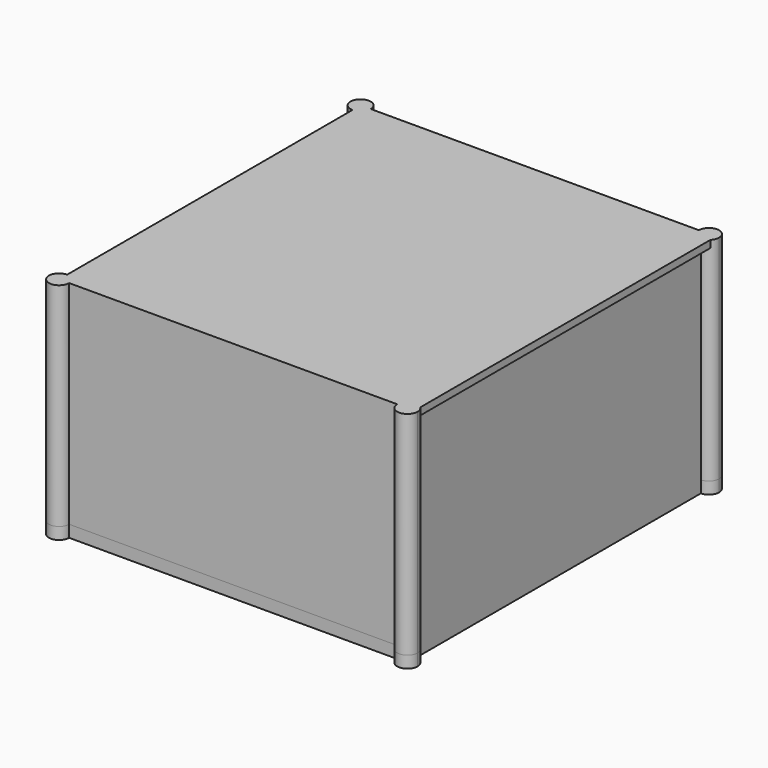
from build123d import *

# Parameters (mm, degrees)
F0_W          = 5
F0_H          = 26
F1_DEPTH      = 5
F2_DEPTH      = 86
F3_DEPTH      = 3
F4_DEPTH      = 89
F5_START      = 86
F5_DEPTH      = 3
F6_R          = 1.925
F7_DEPTH      = 20
F7_DEPTH_BACK = 5
F8_DEPTH      = 3
F9_DEPTH      = 1.2426406871
F10_DEPTH     = 1.2426406871


# Not quite as in the source:
# - a feature names something its author has since deleted; it is built from what else it names


with BuildPart() as f1:
    # F0 (on Top) → F1 (new body)
    with BuildSketch(Plane.XY):
        with BuildLine():
            ThreePointArc((73, 74.7573593129), (71.3764116996, 75.0803111054), (70, 76))
            Line((70, 76), (70, -76))
            ThreePointArc((70, -76), (71.3764116996, -75.0803111054), (73, -74.7573593129))
            Line((73, -74.7573593129), (73, 74.7573593129))
        make_face()
        Polygon((70, -76), (70, 76), (-30, 76), (-30, 50), (-30, -50), (-30, -76), align=None)
        Polygon((-35, 50), (-35, 76), (-70, 76), (-70, -76), (-35, -76), (-35, -50), (-30, -50), (-30, 50), align=None)
        with Locations((-32.5, -63)):
            Rectangle(F0_W, F0_H)
        with Locations((-32.5, 63)):
            Rectangle(F0_W, F0_H)
        with BuildLine():
            Line((-70, -76), (-70, 76))
            ThreePointArc((-70, 76), (-71.3764116996, 75.0803111054), (-73, 74.7573593129))
            Line((-73, 74.7573593129), (-73, -74.7573593129))
            ThreePointArc((-73, -74.7573593129), (-71.3764116996, -75.0803111054), (-70, -76))
        make_face()
        with BuildLine():
            ThreePointArc((73, -74.7573593129), (71.3764116996, -75.0803111054), (70, -76))
            Line((70, -76), (73, -76))
            Line((73, -76), (73, -74.7573593129))
        make_face()
        with BuildLine():
            Line((73, -76), (70, -76))
            ThreePointArc((70, -76), (69.0803111054, -77.3764116996), (68.7573593129, -79))
            Line((68.7573593129, -79), (73, -79))
            Line((73, -79), (73, -76))
        make_face()
        with BuildLine():
            Line((73, -74.7573593129), (73, -76))
            Line((73, -76), (73, -79))
            Line((73, -79), (68.7573593129, -79))
            ThreePointArc((68.7573593129, -79), (73, -83.2426406871), (77.2426406871, -79))
            ThreePointArc((77.2426406871, -79), (76, -76), (73, -74.7573593129))
        make_face()
        with BuildLine():
            Line((73, 76), (70, 76))
            ThreePointArc((70, 76), (71.3764116996, 75.0803111054), (73, 74.7573593129))
            Line((73, 74.7573593129), (73, 76))
        make_face()
        with BuildLine():
            ThreePointArc((68.7573593129, 79), (69.0803111054, 77.3764116996), (70, 76))
            Line((70, 76), (73, 76))
            Line((73, 76), (73, 79))
            Line((73, 79), (68.7573593129, 79))
        make_face()
        with BuildLine():
            Line((73, 79), (73, 76))
            Line((73, 76), (73, 74.7573593129))
            ThreePointArc((73, 74.7573593129), (76, 76), (77.2426406871, 79))
            ThreePointArc((77.2426406871, 79), (73, 83.2426406871), (68.7573593129, 79))
            Line((68.7573593129, 79), (73, 79))
        make_face()
        with BuildLine():
            Line((-30, 76), (70, 76))
            ThreePointArc((70, 76), (69.0803111054, 77.3764116996), (68.7573593129, 79))
            Line((68.7573593129, 79), (-68.7573593129, 79))
            ThreePointArc((-68.7573593129, 79), (-69.0803111054, 77.3764116996), (-70, 76))
            Line((-70, 76), (-35, 76))
            Line((-35, 76), (-30, 76))
        make_face()
        with BuildLine():
            ThreePointArc((-70, 76), (-69.0803111054, 77.3764116996), (-68.7573593129, 79))
            Line((-68.7573593129, 79), (-73, 79))
            Line((-73, 79), (-73, 74.7573593129))
            ThreePointArc((-73, 74.7573593129), (-71.3764116996, 75.0803111054), (-70, 76))
        make_face()
        with BuildLine():
            Line((-73, 79), (-68.7573593129, 79))
            ThreePointArc((-68.7573593129, 79), (-76, 82), (-73, 74.7573593129))
            Line((-73, 74.7573593129), (-73, 79))
        make_face()
        with BuildLine():
            Line((-73, -79), (-68.7573593129, -79))
            ThreePointArc((-68.7573593129, -79), (-69.0803111054, -77.3764116996), (-70, -76))
            ThreePointArc((-70, -76), (-71.3764116996, -75.0803111054), (-73, -74.7573593129))
            Line((-73, -74.7573593129), (-73, -79))
        make_face()
        with BuildLine():
            ThreePointArc((-73, -74.7573593129), (-76, -82), (-68.7573593129, -79))
            Line((-68.7573593129, -79), (-73, -79))
            Line((-73, -79), (-73, -74.7573593129))
        make_face()
        with BuildLine():
            ThreePointArc((68.7573593129, -79), (69.0803111054, -77.3764116996), (70, -76))
            Line((70, -76), (-30, -76))
            Line((-30, -76), (-35, -76))
            Line((-35, -76), (-70, -76))
            ThreePointArc((-70, -76), (-69.0803111054, -77.3764116996), (-68.7573593129, -79))
            Line((-68.7573593129, -79), (68.7573593129, -79))
        make_face()
    extrude(amount=-F1_DEPTH)

    # F0 (on Top) → F2 (join)
    with BuildSketch(Plane.XY):
        with BuildLine():
            ThreePointArc((73, 74.7573593129), (71.3764116996, 75.0803111054), (70, 76))
            Line((70, 76), (70, -76))
            ThreePointArc((70, -76), (71.3764116996, -75.0803111054), (73, -74.7573593129))
            Line((73, -74.7573593129), (73, 74.7573593129))
        make_face()
    extrude(amount=F2_DEPTH)

    # F0 (on Top) → F3 (join)
    with BuildSketch(Plane.XY):
        with Locations((-32.5, 63)):
            Rectangle(F0_W, F0_H)
        with Locations((-32.5, -63)):
            Rectangle(F0_W, F0_H)
    extrude(amount=F3_DEPTH)


with BuildPart() as f4:
    # F0 (on Top) → F4 (new body)
    with BuildSketch(Plane.XY):
        with BuildLine():
            Line((-70, -76), (-70, 76))
            ThreePointArc((-70, 76), (-71.3764116996, 75.0803111054), (-73, 74.7573593129))
            Line((-73, 74.7573593129), (-73, -74.7573593129))
            ThreePointArc((-73, -74.7573593129), (-71.3764116996, -75.0803111054), (-70, -76))
        make_face()
        with BuildLine():
            Line((73, -76), (70, -76))
            ThreePointArc((70, -76), (69.0803111054, -77.3764116996), (68.7573593129, -79))
            Line((68.7573593129, -79), (73, -79))
            Line((73, -79), (73, -76))
        make_face()
        with BuildLine():
            ThreePointArc((68.7573593129, 79), (69.0803111054, 77.3764116996), (70, 76))
            Line((70, 76), (73, 76))
            Line((73, 76), (73, 79))
            Line((73, 79), (68.7573593129, 79))
        make_face()
        with BuildLine():
            Line((73, 79), (73, 76))
            Line((73, 76), (73, 74.7573593129))
            ThreePointArc((73, 74.7573593129), (76, 76), (77.2426406871, 79))
            ThreePointArc((77.2426406871, 79), (73, 83.2426406871), (68.7573593129, 79))
            Line((68.7573593129, 79), (73, 79))
        make_face()
        with BuildLine():
            Line((73, -74.7573593129), (73, -76))
            Line((73, -76), (73, -79))
            Line((73, -79), (68.7573593129, -79))
            ThreePointArc((68.7573593129, -79), (73, -83.2426406871), (77.2426406871, -79))
            ThreePointArc((77.2426406871, -79), (76, -76), (73, -74.7573593129))
        make_face()
        with BuildLine():
            ThreePointArc((73, -74.7573593129), (71.3764116996, -75.0803111054), (70, -76))
            Line((70, -76), (73, -76))
            Line((73, -76), (73, -74.7573593129))
        make_face()
        with BuildLine():
            Line((73, 76), (70, 76))
            ThreePointArc((70, 76), (71.3764116996, 75.0803111054), (73, 74.7573593129))
            Line((73, 74.7573593129), (73, 76))
        make_face()
        with BuildLine():
            Line((-73, -79), (-68.7573593129, -79))
            ThreePointArc((-68.7573593129, -79), (-69.0803111054, -77.3764116996), (-70, -76))
            ThreePointArc((-70, -76), (-71.3764116996, -75.0803111054), (-73, -74.7573593129))
            Line((-73, -74.7573593129), (-73, -79))
        make_face()
        with BuildLine():
            ThreePointArc((68.7573593129, -79), (69.0803111054, -77.3764116996), (70, -76))
            Line((70, -76), (-30, -76))
            Line((-30, -76), (-35, -76))
            Line((-35, -76), (-70, -76))
            ThreePointArc((-70, -76), (-69.0803111054, -77.3764116996), (-68.7573593129, -79))
            Line((-68.7573593129, -79), (68.7573593129, -79))
        make_face()
        with BuildLine():
            ThreePointArc((-73, -74.7573593129), (-76, -82), (-68.7573593129, -79))
            Line((-68.7573593129, -79), (-73, -79))
            Line((-73, -79), (-73, -74.7573593129))
        make_face()
        with BuildLine():
            Line((-30, 76), (70, 76))
            ThreePointArc((70, 76), (69.0803111054, 77.3764116996), (68.7573593129, 79))
            Line((68.7573593129, 79), (-68.7573593129, 79))
            ThreePointArc((-68.7573593129, 79), (-69.0803111054, 77.3764116996), (-70, 76))
            Line((-70, 76), (-35, 76))
            Line((-35, 76), (-30, 76))
        make_face()
        with BuildLine():
            Line((-73, 79), (-68.7573593129, 79))
            ThreePointArc((-68.7573593129, 79), (-76, 82), (-73, 74.7573593129))
            Line((-73, 74.7573593129), (-73, 79))
        make_face()
        with BuildLine():
            ThreePointArc((-70, 76), (-69.0803111054, 77.3764116996), (-68.7573593129, 79))
            Line((-68.7573593129, 79), (-73, 79))
            Line((-73, 79), (-73, 74.7573593129))
            ThreePointArc((-73, 74.7573593129), (-71.3764116996, 75.0803111054), (-70, 76))
        make_face()
    extrude(amount=F4_DEPTH)

    # F0 (on Top) → F5 (join)
    with BuildSketch(Plane.XY.offset(F5_START)):
        Polygon((70, -76), (70, 76), (-30, 76), (-30, 50), (-30, -50), (-30, -76), align=None)
        Polygon((-35, 50), (-35, 76), (-70, 76), (-70, -76), (-35, -76), (-35, -50), (-30, -50), (-30, 50), align=None)
        with Locations((-32.5, 63)):
            Rectangle(F0_W, F0_H)
        with Locations((-32.5, -63)):
            Rectangle(F0_W, F0_H)
        with BuildLine():
            ThreePointArc((73, 74.7573593129), (71.3764116996, 75.0803111054), (70, 76))
            Line((70, 76), (70, -76))
            ThreePointArc((70, -76), (71.3764116996, -75.0803111054), (73, -74.7573593129))
            Line((73, -74.7573593129), (73, 74.7573593129))
        make_face()
        with BuildLine():
            ThreePointArc((73, -74.7573593129), (71.3764116996, -75.0803111054), (70, -76))
            Line((70, -76), (73, -76))
            Line((73, -76), (73, -74.7573593129))
        make_face()
        with BuildLine():
            Line((73, 76), (70, 76))
            ThreePointArc((70, 76), (71.3764116996, 75.0803111054), (73, 74.7573593129))
            Line((73, 74.7573593129), (73, 76))
        make_face()
        with BuildLine():
            ThreePointArc((68.7573593129, 79), (69.0803111054, 77.3764116996), (70, 76))
            Line((70, 76), (73, 76))
            Line((73, 76), (73, 79))
            Line((73, 79), (68.7573593129, 79))
        make_face()
        with BuildLine():
            Line((-70, -76), (-70, 76))
            ThreePointArc((-70, 76), (-71.3764116996, 75.0803111054), (-73, 74.7573593129))
            Line((-73, 74.7573593129), (-73, -74.7573593129))
            ThreePointArc((-73, -74.7573593129), (-71.3764116996, -75.0803111054), (-70, -76))
        make_face()
        with BuildLine():
            Line((73, 79), (73, 76))
            Line((73, 76), (73, 74.7573593129))
            ThreePointArc((73, 74.7573593129), (76, 76), (77.2426406871, 79))
            ThreePointArc((77.2426406871, 79), (73, 83.2426406871), (68.7573593129, 79))
            Line((68.7573593129, 79), (73, 79))
        make_face()
        with BuildLine():
            Line((73, -76), (70, -76))
            ThreePointArc((70, -76), (69.0803111054, -77.3764116996), (68.7573593129, -79))
            Line((68.7573593129, -79), (73, -79))
            Line((73, -79), (73, -76))
        make_face()
        with BuildLine():
            Line((73, -74.7573593129), (73, -76))
            Line((73, -76), (73, -79))
            Line((73, -79), (68.7573593129, -79))
            ThreePointArc((68.7573593129, -79), (73, -83.2426406871), (77.2426406871, -79))
            ThreePointArc((77.2426406871, -79), (76, -76), (73, -74.7573593129))
        make_face()
    extrude(amount=F5_DEPTH)


with BuildPart() as f7_tool:
    # F6 (on Top) → F7 (new body, two sides)
    with BuildSketch(Plane.XY) as f7_sk:
        with Locations((73, -79)):
            Circle(F6_R)
        with Locations((73, 79)):
            Circle(F6_R)
        with Locations((-73, -79)):
            Circle(F6_R)
        with Locations((-73, 79)):
            Circle(F6_R)
    extrude(amount=F7_DEPTH)
    extrude(f7_sk.sketch, amount=-F7_DEPTH_BACK)


with BuildPart() as f1_1:
    add(f1.part)

    # F7: cut by f7_tool
    add(f7_tool.part, mode=Mode.SUBTRACT)


with BuildPart() as f4_1:
    add(f4.part)

    # F7: cut by f7_tool
    add(f7_tool.part, mode=Mode.SUBTRACT)

    # F8 (add): a face of the model
    f8_faces = [f4_1.faces().sort_by_distance(p)[0] for p in [
        (73, 0, 87.5),
    ]]
    extrude(f8_faces, amount=F8_DEPTH)

    # F9 (add, through all): a face of the model
    f9_faces = [f4_1.faces().sort_by_distance(p)[0] for p in [
        (74.5, -74.7573593129, 87.5),
    ]]
    extrude(f9_faces, amount=F9_DEPTH)

    # F10 (add, through all): a face of the model
    f10_faces = [f4_1.faces().sort_by_distance(p)[0] for p in [
        (74.5, 74.7573593129, 87.5),
    ]]
    extrude(f10_faces, amount=F10_DEPTH)


solid = Compound([f1_1.part, f4_1.part])
